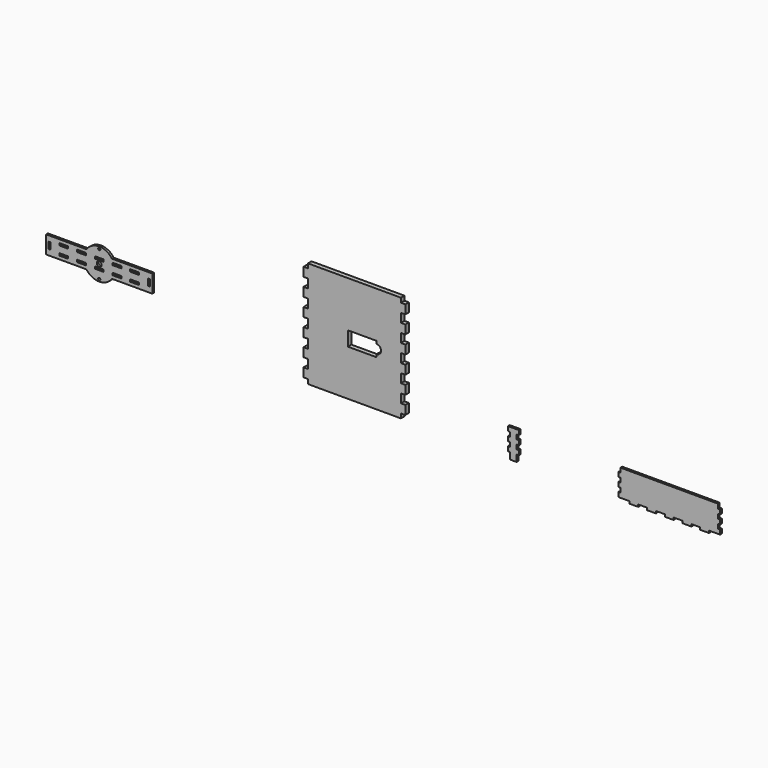
from build123d import *

# Parameters (mm, degrees)
F0_W     = 12.7
F0_H     = 3.175
F1_DEPTH = 3.175
F2_W     = 9.525
F2_H     = 3.175
F2_W_2   = 3.175
F2_H_2   = 6.35
F3_DEPTH = 3.175
F4_W     = 6.35
F4_H     = 12.7
F5_DEPTH = 6.35
F6_R     = 3.4925
F6_R_2   = 1.5875
F7_DEPTH = 3.175
F8_W     = 12.7
F8_H     = 3.175
F8_W_2   = 3.175
F8_H_2   = 9.525
F9_DEPTH = 3.175


with BuildPart() as f1:
    # F0 (on Front) → F1 (new body)
    with BuildSketch(Plane.XZ):
        Polygon((0, 6.35), (0, 0), (15.875, 0), (28.575, 0), (41.275, 0), (53.975, 0), (66.675, 0), (79.375, 0), (92.075, 0), (104.775, 0), (117.475, 0), (130.175, 0), (146.05, 0), (146.05, 6.35), (142.875, 6.35), (142.875, 12.7), (146.05, 12.7), (146.05, 19.05), (142.875, 19.05), (142.875, 25.4), (146.05, 25.4), (146.05, 31.75), (142.875, 31.75), (142.875, 38.1), (3.175, 38.1), (3.175, 31.75), (0, 31.75), (0, 25.4), (3.175, 25.4), (3.175, 19.05), (0, 19.05), (0, 12.7), (3.175, 12.7), (3.175, 6.35), align=None)
        with Locations((22.225, -1.5875)):
            Rectangle(F0_W, F0_H)
        with Locations((47.625, -1.5875)):
            Rectangle(F0_W, F0_H)
        with Locations((73.025, -1.5875)):
            Rectangle(F0_W, F0_H)
        with Locations((98.425, -1.5875)):
            Rectangle(F0_W, F0_H)
        with Locations((123.825, -1.5875)):
            Rectangle(F0_W, F0_H)
    extrude(amount=F1_DEPTH)


with BuildPart() as f3:
    # F2 (on Front) → F3 (new body)
    with BuildSketch(Plane.XZ):
        with Locations((-150.4022690821, -1.5875)):
            Rectangle(F2_W, F2_H)
        Polygon((-155.1647690821, 0), (-145.6397690821, 0), (-145.6397690821, 6.35), (-145.6397690821, 12.7), (-145.6397690821, 19.05), (-145.6397690821, 25.4), (-145.6397690821, 31.75), (-145.6397690821, 38.1), (-155.1647690821, 38.1), (-155.1647690821, 31.75), (-155.1647690821, 25.4), (-155.1647690821, 19.05), (-155.1647690821, 12.7), (-155.1647690821, 6.35), align=None)
        with Locations((-144.0522690821, 9.525)):
            Rectangle(F2_W_2, F2_H_2)
        with Locations((-156.7522690821, 9.525)):
            Rectangle(F2_W_2, F2_H_2)
        with Locations((-144.0522690821, 22.225)):
            Rectangle(F2_W_2, F2_H_2)
        with Locations((-156.7522690821, 22.225)):
            Rectangle(F2_W_2, F2_H_2)
        with Locations((-144.0522690821, 34.925)):
            Rectangle(F2_W_2, F2_H_2)
        with Locations((-156.7522690821, 34.925)):
            Rectangle(F2_W_2, F2_H_2)
    extrude(amount=F3_DEPTH)


with BuildPart() as f5:
    # F4 (on Front) → F5 (new body)
    with BuildSketch(Plane.XZ):
        Polygon((-442.4599377941, 0), (-309.1099377941, 0), (-309.1099377941, 6.35), (-309.1099377941, 19.05), (-309.1099377941, 31.75), (-309.1099377941, 44.45), (-309.1099377941, 57.15), (-309.1099377941, 69.85), (-309.1099377941, 82.55), (-309.1099377941, 95.25), (-309.1099377941, 107.95), (-309.1099377941, 120.65), (-309.1099377941, 133.35), (-309.1099377941, 146.05), (-309.1099377941, 152.4), (-442.4599377941, 152.4), (-442.4599377941, 146.05), (-442.4599377941, 133.35), (-442.4599377941, 127), (-442.4599377941, 120.65), (-442.4599377941, 107.95), (-442.4599377941, 101.6), (-442.4599377941, 95.25), (-442.4599377941, 82.55), (-442.4599377941, 76.2), (-442.4599377941, 69.85), (-442.4599377941, 57.15), (-442.4599377941, 50.8), (-442.4599377941, 44.45), (-442.4599377941, 31.75), (-442.4599377941, 19.05), (-442.4599377941, 6.35), align=None)
        with BuildLine():
            Line((-385.3099377941, 65.85), (-385.3099377941, 86.55))
            Line((-385.3099377941, 86.55), (-344.0099377941, 86.55))
            Line((-344.0099377941, 86.55), (-344.0099377941, 82.55))
            ThreePointArc((-344.0099377941, 82.55), (-339.5198097336, 80.6901280605), (-337.6599377941, 76.2))
            ThreePointArc((-337.6599377941, 76.2), (-339.5198097336, 71.7098719395), (-344.0099377941, 69.85))
            Line((-344.0099377941, 69.85), (-344.0099377941, 65.85))
            Line((-344.0099377941, 65.85), (-385.3099377941, 65.85))
        make_face(mode=Mode.SUBTRACT)
        with Locations((-305.9349377941, 12.7)):
            Rectangle(F4_W, F4_H)
        with Locations((-445.6349377941, 12.7)):
            Rectangle(F4_W, F4_H)
        with Locations((-305.9349377941, 38.1)):
            Rectangle(F4_W, F4_H)
        with Locations((-445.6349377941, 38.1)):
            Rectangle(F4_W, F4_H)
        with Locations((-305.9349377941, 63.5)):
            Rectangle(F4_W, F4_H)
        with Locations((-445.6349377941, 63.5)):
            Rectangle(F4_W, F4_H)
        with Locations((-305.9349377941, 88.9)):
            Rectangle(F4_W, F4_H)
        with Locations((-305.9349377941, 114.3)):
            Rectangle(F4_W, F4_H)
        with Locations((-445.6349377941, 88.9)):
            Rectangle(F4_W, F4_H)
        with Locations((-305.9349377941, 139.7)):
            Rectangle(F4_W, F4_H)
        with Locations((-445.6349377941, 114.3)):
            Rectangle(F4_W, F4_H)
        with Locations((-445.6349377941, 139.7)):
            Rectangle(F4_W, F4_H)
    extrude(amount=F5_DEPTH)


with BuildPart() as f7:
    # F6 (on Front) → F7 (new body)
    with BuildSketch(Plane.XZ):
        with BuildLine():
            ThreePointArc((-726.009471792, 39.3724814057), (-723.043363314, 45.4170643565), (-722.0234581947, 52.0724814057))
            ThreePointArc((-722.0234581947, 52.0724814057), (-723.043363314, 58.727898455), (-726.009471792, 64.7724814057))
            Line((-726.009471792, 64.7724814057), (-762.4874445975, 64.7724814057))
            ThreePointArc((-762.4874445975, 64.7724814057), (-766.4734581947, 52.0724814057), (-762.4874445975, 39.3724814057))
            Line((-762.4874445975, 39.3724814057), (-726.009471792, 39.3724814057))
        make_face()
        with Locations((-744.2484581947, 52.0724814057)):
            Circle(F6_R, mode=Mode.SUBTRACT)
        with BuildLine():
            ThreePointArc((-762.4874445975, 39.3724814057), (-766.4734581947, 52.0724814057), (-762.4874445975, 64.7724814057))
            Line((-762.4874445975, 64.7724814057), (-820.4484581947, 64.7724814057))
            Line((-820.4484581947, 64.7724814057), (-820.4484581947, 39.3724814057))
            Line((-820.4484581947, 39.3724814057), (-762.4874445975, 39.3724814057))
        make_face()
        with BuildLine():
            ThreePointArc((-726.009471792, 64.7724814057), (-723.043363314, 58.727898455), (-722.0234581947, 52.0724814057))
            ThreePointArc((-722.0234581947, 52.0724814057), (-723.043363314, 45.4170643565), (-726.009471792, 39.3724814057))
            Line((-726.009471792, 39.3724814057), (-668.0484581947, 39.3724814057))
            Line((-668.0484581947, 39.3724814057), (-668.0484581947, 64.7724814057))
            Line((-668.0484581947, 64.7724814057), (-726.009471792, 64.7724814057))
        make_face()
        with BuildLine():
            Line((-762.4874445975, 64.7724814057), (-726.009471792, 64.7724814057))
            ThreePointArc((-726.009471792, 64.7724814057), (-744.2484581947, 74.2974814057), (-762.4874445975, 64.7724814057))
        make_face()
        with Locations((-744.2484581947, 71.1224814057)):
            Circle(F6_R_2, mode=Mode.SUBTRACT)
        with BuildLine():
            ThreePointArc((-762.4874445975, 39.3724814057), (-744.2484581947, 29.8474814057), (-726.009471792, 39.3724814057))
            Line((-726.009471792, 39.3724814057), (-762.4874445975, 39.3724814057))
        make_face()
        with Locations((-744.2484581947, 33.0224814057)):
            Circle(F6_R_2, mode=Mode.SUBTRACT)
    extrude(amount=F7_DEPTH)

    # F8 (on face) → F9 (cut, through all)
    with BuildSketch(Plane.XZ.offset(3.175)):
        with Locations((-744.2484581947, 58.4224814057)):
            Rectangle(F8_W, F8_H)
        with Locations((-769.6484581947, 58.4224814057)):
            Rectangle(F8_W, F8_H)
        with Locations((-795.0484581947, 58.4224814057)):
            Rectangle(F8_W, F8_H)
        with Locations((-718.8484581947, 58.4224814057)):
            Rectangle(F8_W, F8_H)
        with Locations((-693.4484581947, 58.4224814057)):
            Rectangle(F8_W, F8_H)
        with Locations((-744.2484581947, 45.7224814057)):
            Rectangle(F8_W, F8_H)
        with Locations((-769.6484581947, 45.7224814057)):
            Rectangle(F8_W, F8_H)
        with Locations((-718.8484581947, 45.7224814057)):
            Rectangle(F8_W, F8_H)
        with Locations((-795.0484581947, 45.7224814057)):
            Rectangle(F8_W, F8_H)
        with Locations((-693.4484581947, 45.7224814057)):
            Rectangle(F8_W, F8_H)
        with Locations((-815.6859581947, 52.0724814057)):
            Rectangle(F8_W_2, F8_H_2)
        with Locations((-672.8109581947, 52.0724814057)):
            Rectangle(F8_W_2, F8_H_2)
    extrude(amount=-F9_DEPTH, mode=Mode.SUBTRACT)


solid = Compound([f1.part, f3.part, f5.part, f7.part])
